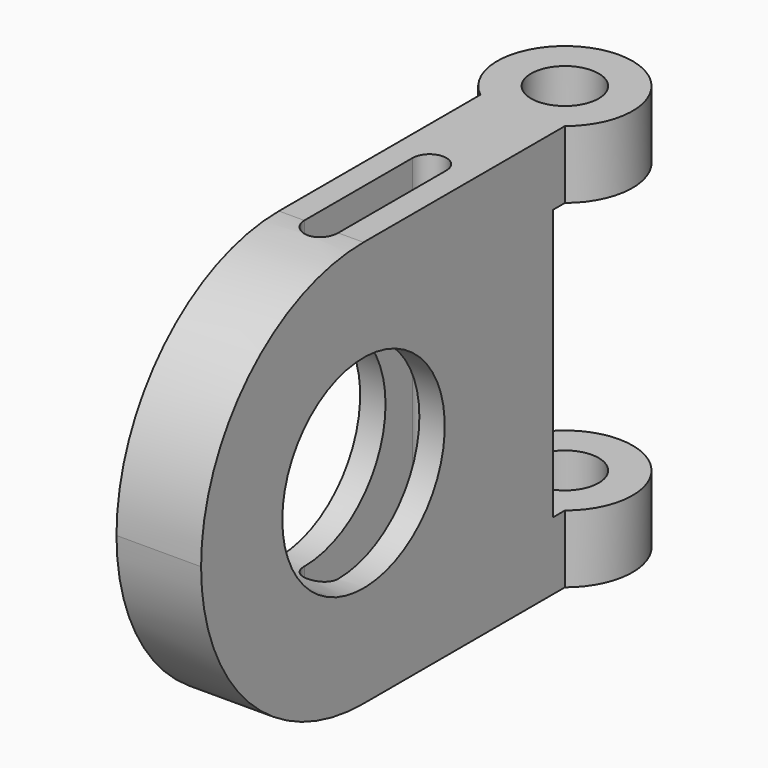
from build123d import *

# Parameters (mm, degrees)
F0_R     = 12.7
F1_DEPTH = 152.4
F2_R     = 76.19999
F3_R     = 38.1
F3_W     = 84.1318353355
F3_H     = 101.6
F4_DEPTH = 6350
F6_DEPTH = 241.62033
F5_R     = 12.7
F7_DEPTH = 170.20256


# Not quite as in the source:
# - a fillet or chamfer is up to 0.001 mm smaller than in the source, because OpenCascade refuses the exact size
# - ends of sketch curves that miss each other by under 0.0002 mm in the source are joined


with BuildPart() as f1:
    # F0 (on Top) → F1 (new body)
    with BuildSketch(Plane.XY):
        with BuildLine():
            Line((15.875, -190.5), (15.875, -19.8278686449))
            ThreePointArc((15.875, -19.8278686449), (0, 25.4), (-15.875, -19.8278686449))
            Line((-15.875, -19.8278686449), (-15.875, -190.5))
            Line((-15.875, -190.5), (15.875, -190.5))
        make_face()
        Circle(F0_R, mode=Mode.SUBTRACT)
    extrude(amount=F1_DEPTH)

    # F2 (radius 76.2 in the source; OpenCascade refuses exactly that, so slightly less here)
    f2_edges = [f1.edges().sort_by_distance(p)[0] for p in [
        (0, -190.5, 152.4),
        (0, -190.5, 0),
    ]]
    fillet(f2_edges, radius=F2_R)

    # F3 (on face) → F4 (cut, symmetric)
    with BuildSketch(Plane(origin=(-15.875, 0, 0), x_dir=(0, -1, 0), z_dir=(-1, 0, 0))):
        with Locations((114.3, 76.2)):
            Circle(F3_R)
        with Locations((-16.6659176677, 76.2)):
            Rectangle(F3_W, F3_H)
    extrude(amount=F4_DEPTH, both=True, mode=Mode.SUBTRACT)

    # F5 (on face) → F6 (cut, symmetric)
    with BuildSketch(Plane.XY.offset(152.4)):
        with BuildLine():
            ThreePointArc((6.35, -63.5), (0, -57.15), (-6.35, -63.5))
            Line((-6.35, -63.5), (-6.35, -114.3))
            Line((-6.35, -114.3), (6.35, -114.30001))
            Line((6.35, -114.30001), (6.35, -63.5))
        make_face()
    extrude(amount=F6_DEPTH, both=True, mode=Mode.SUBTRACT)

    # F5 (on face) → F7 (cut)
    with BuildSketch(Plane.XY.offset(152.4)):
        Circle(F5_R)
        with BuildLine():
            ThreePointArc((6.35, -63.5), (0, -57.15), (-6.35, -63.5))
            Line((-6.35, -63.5), (-6.35, -114.3))
            ThreePointArc((-6.35, -114.3), (0, -120.65), (6.35, -114.3))
            Line((6.35, -114.3), (6.35, -63.5))
        make_face()
    extrude(amount=-F7_DEPTH, mode=Mode.SUBTRACT)


solid = f1.part
